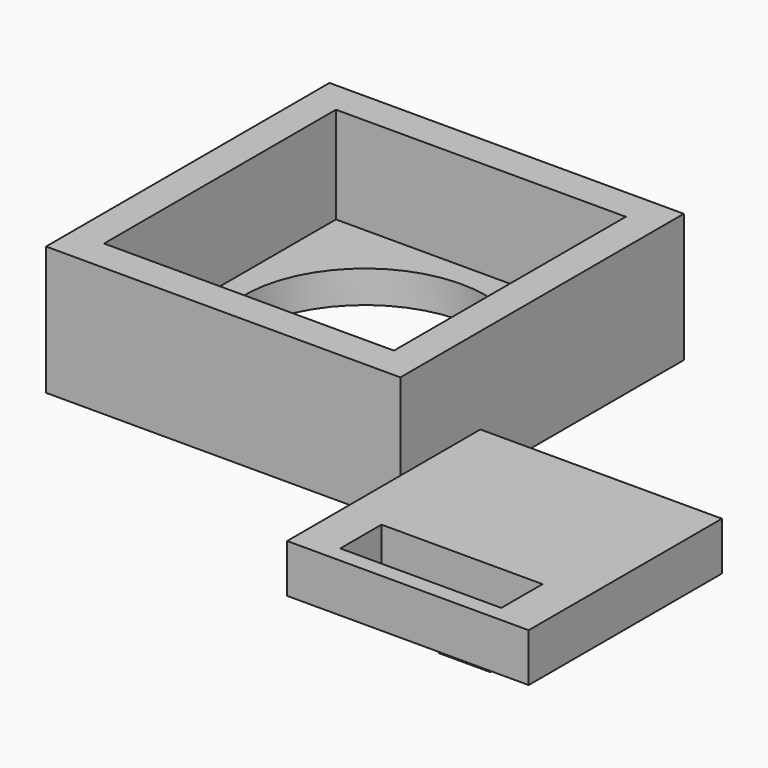
from build123d import *

# Parameters (mm, degrees)
F0_W       = 22
F0_H       = 22
F0_W_2     = 18
F0_H_2     = 18
F0_R       = 7.5
F1_DEPTH   = 2
F2_DEPTH   = 6
F5_W       = 15
F5_H       = 15
F5_W_2     = 10
F5_H_2     = 3.2
F13_DEPTH  = 3
F7_W       = 3.2
F7_H       = 1
F7_W_2     = 1
F7_H_2     = 3.2
F14_DEPTH  = 2
F14_FACE_W = 1
F14_FACE_H = 3.2
F10_W      = 1.6
F10_H      = 3.2
F17_DEPTH  = 0.5
F15_FACE_W = 1.6
F15_FACE_H = 3.2
F12_W      = 1
F12_H      = 3.2
F16_FACE_W = 1.6
F16_FACE_H = 3.2
F20_DEPTH  = 0.5


# Not quite as in the source:
# - a feature names something its author has since deleted; it is built from what else it names


with BuildPart() as f1:
    # F0 (on Top) → F1 (new body)
    with BuildSketch(Plane.XY):
        with Locations((-35.0640561283, 11.6431117058)):
            Rectangle(F0_W, F0_H)
        with Locations((-35.0640561283, 11.6431117058)):
            Rectangle(F0_W_2, F0_H_2, mode=Mode.SUBTRACT)
        with Locations((-35.0640561283, 11.6431117058)):
            Rectangle(F0_W_2, F0_H_2)
        with Locations((-35.0640561283, 11.6431117058)):
            Circle(F0_R, mode=Mode.SUBTRACT)
    extrude(amount=-F1_DEPTH)

    # F0 (on Top) → F2 (join)
    with BuildSketch(Plane.XY):
        with Locations((-35.0640561283, 11.6431117058)):
            Rectangle(F0_W, F0_H)
        with Locations((-35.0640561283, 11.6431117058)):
            Rectangle(F0_W_2, F0_H_2, mode=Mode.SUBTRACT)
    extrude(amount=F2_DEPTH)


with BuildPart() as f13:
    # F5 (on offset) → F13 (new body, through all)
    with BuildSketch(Plane.XY.offset(10)):
        with Locations((-5.3186413549, -14.7037236601)):
            Rectangle(F5_W, F5_H)
        with Locations((-5.3186413549, -19.6037236601)):
            Rectangle(F5_W_2, F5_H_2, mode=Mode.SUBTRACT)
    extrude(amount=-F13_DEPTH)

    # F7 (on offset) → F14 (join, through all)
    with BuildSketch(Plane.XY.offset(7)):
        with Locations((-5.3186413549, -12.1037236601)):
            Rectangle(F7_W, F7_H)
        with Locations((-2.7186413549, -14.7037236601)):
            Rectangle(F7_W_2, F7_H_2)
        with Locations((-5.3186413549, -17.3037236601)):
            Rectangle(F7_W, F7_H)
        with Locations((-7.9186413549, -14.7037236601)):
            Rectangle(F7_W_2, F7_H_2)
    extrude(amount=-F14_DEPTH)

    # F14_face (on face) → F15 section 0
    with BuildSketch(Plane(origin=(-2.7186413549, -14.7037236601, 5), x_dir=(1, 0, 0), z_dir=(0, 0, -1))):
        Rectangle(F14_FACE_W, F14_FACE_H)
    # F10 (on offset) → F15 section 1
    with BuildSketch(Plane.XY.offset(4.5)):
        with Locations((-3.0186413549, -14.7037236601)):
            Rectangle(F10_W, F10_H)
    loft()

    # F14_face (on face) → F16 section 0
    with BuildSketch(Plane(origin=(-2.7186413549, -14.7037236601, 5), x_dir=(1, 0, 0), z_dir=(0, 0, -1))):
        with Locations((-5.2, 0)):
            Rectangle(F14_FACE_W, F14_FACE_H)
    # F10 (on offset) → F16 section 1
    with BuildSketch(Plane.XY.offset(4.5)):
        with Locations((-7.6186413549, -14.7037236601)):
            Rectangle(F10_W, F10_H)
    loft()

    # F17 (add, through all): faces of the model
    f17_faces = [f13.faces().sort_by_distance(p)[0] for p in [
        (-5.3186413549, -12.1037236601, 5),
        (-5.3186413549, -17.3037236601, 5),
    ]]
    extrude(f17_faces, amount=F17_DEPTH)

    # F15_face (on face) → F18 section 0
    with BuildSketch(Plane(origin=(-3.0186413549, -14.7037236601, 4.5), x_dir=(1, 0, 0), z_dir=(0, 0, -1))):
        Rectangle(F15_FACE_W, F15_FACE_H)
    # F12 (on offset) → F18 section 1
    with BuildSketch(Plane.XY.offset(4)):
        with Locations((-2.7186413549, -14.7037236601)):
            Rectangle(F12_W, F12_H)
    loft()

    # F16_face (on face) → F19 section 0
    with BuildSketch(Plane(origin=(-7.6186413549, -14.7037236601, 4.5), x_dir=(1, 0, 0), z_dir=(0, 0, -1))):
        Rectangle(F16_FACE_W, F16_FACE_H)
    # F12 (on offset) → F19 section 1
    with BuildSketch(Plane.XY.offset(4)):
        with Locations((-7.9186413549, -14.7037236601)):
            Rectangle(F12_W, F12_H)
    loft()

    # F20 (add, through all): faces of the model
    f20_faces = [f13.faces().sort_by_distance(p)[0] for p in [
        (-5.3186413549, -17.3037236601, 4.5),
        (-5.3186413549, -12.1037236601, 4.5),
    ]]
    extrude(f20_faces, amount=F20_DEPTH)


solid = Compound([f1.part, f13.part])
